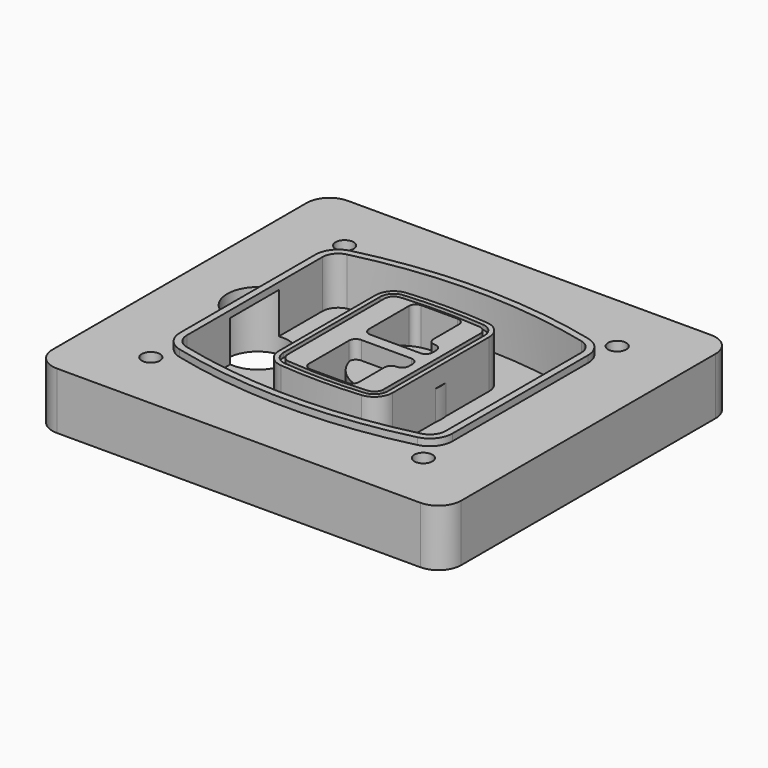
from build123d import *

# Parameters (mm, degrees)
F0_R      = 4
F1_DEPTH  = 25
F2_DEPTH  = 3
F3_DEPTH  = 18
F5_DEPTH  = 21
F6_DEPTH  = 2
F8_DEPTH  = 20
F9_DEPTH  = 16
F10_DEPTH = 25
F7_R      = 6
F7_R_2    = 4
F11_DEPTH = 6


# Not quite as in the source:
# - a feature of the source that left no trace in its solid (it failed there, or was rolled back) is left out


with BuildPart() as f1:
    # F0 (on Top) → F1 (new body)
    with BuildSketch(Plane.XY):
        with BuildLine():
            ThreePointArc((-90, -70), (-87.0710678119, -77.0710678119), (-80, -80))
            Line((-80, -80), (80, -80))
            ThreePointArc((80, -80), (87.0710678119, -77.0710678119), (90, -70))
            Line((90, -70), (90, 70))
            ThreePointArc((90, 70), (87.0710678119, 77.0710678119), (80, 80))
            Line((80, 80), (-80, 80))
            ThreePointArc((-80, 80), (-87.0710678119, 77.0710678119), (-90, 70))
            Line((-90, 70), (-90, -70))
        make_face()
        with Locations((-60, -53.3333333333)):
            Circle(F0_R, mode=Mode.SUBTRACT)
        with Locations((60, -53.3333333333)):
            Circle(F0_R, mode=Mode.SUBTRACT)
        with Locations((-60, 53.3333333333)):
            Circle(F0_R, mode=Mode.SUBTRACT)
        with BuildLine():
            ThreePointArc((-64, 37.2990447398), (-61.0143011354, 45.9411029726), (-53.3306899286, 50.8970778549))
            ThreePointArc((-53.3306899286, 50.8970778549), (0, 57.3333333333), (53.3306899286, 50.8970778549))
            ThreePointArc((53.3306899286, 50.8970778549), (61.0143011354, 45.9411029726), (64, 37.2990447398))
            Line((64, 37.2990447398), (64, -37.2990447398))
            ThreePointArc((64, -37.2990447398), (61.0143011354, -45.9411029726), (53.3306899286, -50.8970778549))
            ThreePointArc((53.3306899286, -50.8970778549), (0, -57.3333333333), (-53.3306899286, -50.8970778549))
            ThreePointArc((-53.3306899286, -50.8970778549), (-61.0143011354, -45.9411029726), (-64, -37.2990447398))
            Line((-64, -37.2990447398), (-64, 37.2990447398))
        make_face(mode=Mode.SUBTRACT)
        with Locations((60, 53.3333333333)):
            Circle(F0_R, mode=Mode.SUBTRACT)
        with BuildLine():
            ThreePointArc((53.3306899286, 50.8970778549), (0, 57.3333333333), (-53.3306899286, 50.8970778549))
            ThreePointArc((-53.3306899286, 50.8970778549), (-61.0143011354, 45.9411029726), (-64, 37.2990447398))
            Line((-64, 37.2990447398), (-64, -37.2990447398))
            ThreePointArc((-64, -37.2990447398), (-61.0143011354, -45.9411029726), (-53.3306899286, -50.8970778549))
            ThreePointArc((-53.3306899286, -50.8970778549), (0, -57.3333333333), (53.3306899286, -50.8970778549))
            ThreePointArc((53.3306899286, -50.8970778549), (61.0143011354, -45.9411029726), (64, -37.2990447398))
            Line((64, -37.2990447398), (64, 37.2990447398))
            ThreePointArc((64, 37.2990447398), (61.0143011354, 45.9411029726), (53.3306899286, 50.8970778549))
        make_face()
        with BuildLine():
            Line((-60, -37.2990447398), (-60, 37.2990447398))
            ThreePointArc((-60, 37.2990447398), (-57.8673579538, 43.4719434775), (-52.3790642347, 47.0119255363))
            ThreePointArc((-52.3790642347, 47.0119255363), (0, 53.3333333333), (52.3790642347, 47.0119255363))
            ThreePointArc((52.3790642347, 47.0119255363), (57.8673579538, 43.4719434775), (60, 37.2990447398))
            Line((60, 37.2990447398), (60, -37.2990447398))
            ThreePointArc((60, -37.2990447398), (57.8673579538, -43.4719434775), (52.3790642347, -47.0119255363))
            ThreePointArc((52.3790642347, -47.0119255363), (0, -53.3333333333), (-52.3790642347, -47.0119255363))
            ThreePointArc((-52.3790642347, -47.0119255363), (-57.8673579538, -43.4719434775), (-60, -37.2990447398))
        make_face(mode=Mode.SUBTRACT)
        with BuildLine():
            ThreePointArc((-52.3790642347, 47.0119255363), (-57.8673579538, 43.4719434775), (-60, 37.2990447398))
            Line((-60, 37.2990447398), (-60, -37.2990447398))
            ThreePointArc((-60, -37.2990447398), (-57.8673579538, -43.4719434775), (-52.3790642347, -47.0119255363))
            ThreePointArc((-52.3790642347, -47.0119255363), (0, -53.3333333333), (52.3790642347, -47.0119255363))
            ThreePointArc((52.3790642347, -47.0119255363), (57.8673579538, -43.4719434775), (60, -37.2990447398))
            Line((60, -37.2990447398), (60, 37.2990447398))
            ThreePointArc((60, 37.2990447398), (57.8673579538, 43.4719434775), (52.3790642347, 47.0119255363))
            ThreePointArc((52.3790642347, 47.0119255363), (0, 53.3333333333), (-52.3790642347, 47.0119255363))
        make_face()
        with BuildLine():
            ThreePointArc((51.6653449643, 44.0980612973), (55.5071505677, 41.6200738562), (57, 37.2990447398))
            Line((57, 37.2990447398), (57, -37.2990447398))
            ThreePointArc((57, -37.2990447398), (55.5071505677, -41.6200738562), (51.6653449643, -44.0980612973))
            ThreePointArc((51.6653449643, -44.0980612973), (0, -50.3333333333), (-51.6653449643, -44.0980612973))
            ThreePointArc((-51.6653449643, -44.0980612973), (-55.5071505677, -41.6200738562), (-57, -37.2990447398))
            Line((-57, -37.2990447398), (-57, 37.2990447398))
            ThreePointArc((-57, 37.2990447398), (-55.5071505677, 41.6200738562), (-51.6653449643, 44.0980612973))
            ThreePointArc((-51.6653449643, 44.0980612973), (0, 50.3333333333), (51.6653449643, 44.0980612973))
        make_face(mode=Mode.SUBTRACT)
        with BuildLine():
            Line((57, -37.2990447398), (57, 37.2990447398))
            ThreePointArc((57, 37.2990447398), (55.5071505677, 41.6200738562), (51.6653449643, 44.0980612973))
            ThreePointArc((51.6653449643, 44.0980612973), (0, 50.3333333333), (-51.6653449643, 44.0980612973))
            ThreePointArc((-51.6653449643, 44.0980612973), (-55.5071505677, 41.6200738562), (-57, 37.2990447398))
            Line((-57, 37.2990447398), (-57, -37.2990447398))
            ThreePointArc((-57, -37.2990447398), (-55.5071505677, -41.6200738562), (-51.6653449643, -44.0980612973))
            ThreePointArc((-51.6653449643, -44.0980612973), (0, -50.3333333333), (51.6653449643, -44.0980612973))
            ThreePointArc((51.6653449643, -44.0980612973), (55.5071505677, -41.6200738562), (57, -37.2990447398))
        make_face()
    extrude(amount=-F1_DEPTH)

    # F0 (on Top) → F2 (join)
    with BuildSketch(Plane.XY):
        with BuildLine():
            ThreePointArc((-52.3790642347, 47.0119255363), (-57.8673579538, 43.4719434775), (-60, 37.2990447398))
            Line((-60, 37.2990447398), (-60, -37.2990447398))
            ThreePointArc((-60, -37.2990447398), (-57.8673579538, -43.4719434775), (-52.3790642347, -47.0119255363))
            ThreePointArc((-52.3790642347, -47.0119255363), (0, -53.3333333333), (52.3790642347, -47.0119255363))
            ThreePointArc((52.3790642347, -47.0119255363), (57.8673579538, -43.4719434775), (60, -37.2990447398))
            Line((60, -37.2990447398), (60, 37.2990447398))
            ThreePointArc((60, 37.2990447398), (57.8673579538, 43.4719434775), (52.3790642347, 47.0119255363))
            ThreePointArc((52.3790642347, 47.0119255363), (0, 53.3333333333), (-52.3790642347, 47.0119255363))
        make_face()
        with BuildLine():
            ThreePointArc((51.6653449643, 44.0980612973), (55.5071505677, 41.6200738562), (57, 37.2990447398))
            Line((57, 37.2990447398), (57, -37.2990447398))
            ThreePointArc((57, -37.2990447398), (55.5071505677, -41.6200738562), (51.6653449643, -44.0980612973))
            ThreePointArc((51.6653449643, -44.0980612973), (0, -50.3333333333), (-51.6653449643, -44.0980612973))
            ThreePointArc((-51.6653449643, -44.0980612973), (-55.5071505677, -41.6200738562), (-57, -37.2990447398))
            Line((-57, -37.2990447398), (-57, 37.2990447398))
            ThreePointArc((-57, 37.2990447398), (-55.5071505677, 41.6200738562), (-51.6653449643, 44.0980612973))
            ThreePointArc((-51.6653449643, 44.0980612973), (0, 50.3333333333), (51.6653449643, 44.0980612973))
        make_face(mode=Mode.SUBTRACT)
    extrude(amount=F2_DEPTH)

    # F0 (on Top) → F3 (cut)
    with BuildSketch(Plane.XY):
        with BuildLine():
            Line((57, -37.2990447398), (57, 37.2990447398))
            ThreePointArc((57, 37.2990447398), (55.5071505677, 41.6200738562), (51.6653449643, 44.0980612973))
            ThreePointArc((51.6653449643, 44.0980612973), (0, 50.3333333333), (-51.6653449643, 44.0980612973))
            ThreePointArc((-51.6653449643, 44.0980612973), (-55.5071505677, 41.6200738562), (-57, 37.2990447398))
            Line((-57, 37.2990447398), (-57, -37.2990447398))
            ThreePointArc((-57, -37.2990447398), (-55.5071505677, -41.6200738562), (-51.6653449643, -44.0980612973))
            ThreePointArc((-51.6653449643, -44.0980612973), (0, -50.3333333333), (51.6653449643, -44.0980612973))
            ThreePointArc((51.6653449643, -44.0980612973), (55.5071505677, -41.6200738562), (57, -37.2990447398))
        make_face()
    extrude(amount=-F3_DEPTH, mode=Mode.SUBTRACT)

    # F4 (on face) → F5 (join, through all)
    with BuildSketch(Plane.XY.offset(3)):
        with BuildLine():
            ThreePointArc((-25, -26.587695628), (-22.8992979869, -31.9912392117), (-17.7004291845, -34.5569740744))
            ThreePointArc((-17.7004291845, -34.5569740744), (0, -35.3333333333), (17.7004291845, -34.5569740744))
            ThreePointArc((17.7004291845, -34.5569740744), (22.8992979869, -31.9912392117), (25, -26.587695628))
            Line((25, -26.587695628), (25, 26.587695628))
            ThreePointArc((25, 26.587695628), (22.8992979869, 31.9912392117), (17.7004291845, 34.5569740744))
            ThreePointArc((17.7004291845, 34.5569740744), (0, 35.3333333333), (-17.7004291845, 34.5569740744))
            ThreePointArc((-17.7004291845, 34.5569740744), (-22.8992979869, 31.9912392117), (-25, 26.587695628))
            Line((-25, 26.587695628), (-25, -26.587695628))
        make_face()
        with BuildLine():
            ThreePointArc((17.5253218884, 32.5646544628), (21.4244734902, 30.6403533158), (23, 26.587695628))
            Line((23, 26.587695628), (23, -26.587695628))
            ThreePointArc((23, -26.587695628), (21.4244734902, -30.6403533158), (17.5253218884, -32.5646544628))
            ThreePointArc((17.5253218884, -32.5646544628), (0, -33.3333333333), (-17.5253218884, -32.5646544628))
            ThreePointArc((-17.5253218884, -32.5646544628), (-21.4244734902, -30.6403533158), (-23, -26.587695628))
            Line((-23, -26.587695628), (-23, 26.587695628))
            ThreePointArc((-23, 26.587695628), (-21.4244734902, 30.6403533158), (-17.5253218884, 32.5646544628))
            ThreePointArc((-17.5253218884, 32.5646544628), (0, 33.3333333333), (17.5253218884, 32.5646544628))
        make_face(mode=Mode.SUBTRACT)
        with BuildLine():
            Line((23, -26.587695628), (23, 26.587695628))
            ThreePointArc((23, 26.587695628), (21.4244734902, 30.6403533158), (17.5253218884, 32.5646544628))
            ThreePointArc((17.5253218884, 32.5646544628), (0, 33.3333333333), (-17.5253218884, 32.5646544628))
            ThreePointArc((-17.5253218884, 32.5646544628), (-21.4244734902, 30.6403533158), (-23, 26.587695628))
            Line((-23, 26.587695628), (-23, -26.587695628))
            ThreePointArc((-23, -26.587695628), (-21.4244734902, -30.6403533158), (-17.5253218884, -32.5646544628))
            ThreePointArc((-17.5253218884, -32.5646544628), (0, -33.3333333333), (17.5253218884, -32.5646544628))
            ThreePointArc((17.5253218884, -32.5646544628), (21.4244734902, -30.6403533158), (23, -26.587695628))
        make_face()
        with BuildLine():
            ThreePointArc((17.3502145923, 30.5723348512), (19.9496489934, 29.2894674198), (21, 26.587695628))
            Line((21, 26.587695628), (21, -26.587695628))
            ThreePointArc((21, -26.587695628), (19.9496489934, -29.2894674198), (17.3502145923, -30.5723348512))
            ThreePointArc((17.3502145923, -30.5723348512), (0, -31.3333333333), (-17.3502145923, -30.5723348512))
            ThreePointArc((-17.3502145923, -30.5723348512), (-19.9496489934, -29.2894674198), (-21, -26.587695628))
            Line((-21, -26.587695628), (-21, 26.587695628))
            ThreePointArc((-21, 26.587695628), (-19.9496489934, 29.2894674198), (-17.3502145923, 30.5723348512))
            ThreePointArc((-17.3502145923, 30.5723348512), (0, 31.3333333333), (17.3502145923, 30.5723348512))
        make_face(mode=Mode.SUBTRACT)
        with BuildLine():
            Line((21, -26.587695628), (21, 26.587695628))
            ThreePointArc((21, 26.587695628), (19.9496489934, 29.2894674198), (17.3502145923, 30.5723348512))
            ThreePointArc((17.3502145923, 30.5723348512), (0, 31.3333333333), (-17.3502145923, 30.5723348512))
            ThreePointArc((-17.3502145923, 30.5723348512), (-19.9496489934, 29.2894674198), (-21, 26.587695628))
            Line((-21, 26.587695628), (-21, -26.587695628))
            ThreePointArc((-21, -26.587695628), (-19.9496489934, -29.2894674198), (-17.3502145923, -30.5723348512))
            ThreePointArc((-17.3502145923, -30.5723348512), (0, -31.3333333333), (17.3502145923, -30.5723348512))
            ThreePointArc((17.3502145923, -30.5723348512), (19.9496489934, -29.2894674198), (21, -26.587695628))
        make_face()
        with BuildLine():
            Line((-8, -2.5), (14, -2.5))
            ThreePointArc((14, -2.5), (16.1213203436, -3.3786796564), (17, -5.5))
            Line((17, -5.5), (17, -7.5))
            ThreePointArc((17, -7.5), (16.1213203436, -9.6213203436), (14, -10.5))
            ThreePointArc((14, -10.5), (11.8786796564, -11.3786796564), (11, -13.5))
            Line((11, -13.5), (11, -27.5))
            ThreePointArc((11, -27.5), (10.1213203436, -29.6213203436), (8, -30.5))
            Line((8, -30.5), (-8, -30.5))
            ThreePointArc((-8, -30.5), (-10.1213203436, -29.6213203436), (-11, -27.5))
            Line((-11, -27.5), (-11, -5.5))
            ThreePointArc((-11, -5.5), (-10.1213203436, -3.3786796564), (-8, -2.5))
        make_face(mode=Mode.SUBTRACT)
        with BuildLine():
            ThreePointArc((-8, 2.5), (-10.1213203436, 3.3786796564), (-11, 5.5))
            Line((-11, 5.5), (-11, 27.5))
            ThreePointArc((-11, 27.5), (-10.1213203436, 29.6213203436), (-8, 30.5))
            Line((-8, 30.5), (8, 30.5))
            ThreePointArc((8, 30.5), (10.1213203436, 29.6213203436), (11, 27.5))
            Line((11, 27.5), (11, 13.5))
            ThreePointArc((11, 13.5), (11.8786796564, 11.3786796564), (14, 10.5))
            ThreePointArc((14, 10.5), (16.1213203436, 9.6213203436), (17, 7.5))
            Line((17, 7.5), (17, 5.5))
            ThreePointArc((17, 5.5), (16.1213203436, 3.3786796564), (14, 2.5))
            Line((14, 2.5), (-8, 2.5))
        make_face(mode=Mode.SUBTRACT)
    extrude(amount=-F5_DEPTH)

    # F4 (on face) → F6 (cut)
    with BuildSketch(Plane.XY.offset(3)):
        with BuildLine():
            Line((23, -26.587695628), (23, 26.587695628))
            ThreePointArc((23, 26.587695628), (21.4244734902, 30.6403533158), (17.5253218884, 32.5646544628))
            ThreePointArc((17.5253218884, 32.5646544628), (0, 33.3333333333), (-17.5253218884, 32.5646544628))
            ThreePointArc((-17.5253218884, 32.5646544628), (-21.4244734902, 30.6403533158), (-23, 26.587695628))
            Line((-23, 26.587695628), (-23, -26.587695628))
            ThreePointArc((-23, -26.587695628), (-21.4244734902, -30.6403533158), (-17.5253218884, -32.5646544628))
            ThreePointArc((-17.5253218884, -32.5646544628), (0, -33.3333333333), (17.5253218884, -32.5646544628))
            ThreePointArc((17.5253218884, -32.5646544628), (21.4244734902, -30.6403533158), (23, -26.587695628))
        make_face()
        with BuildLine():
            ThreePointArc((17.3502145923, 30.5723348512), (19.9496489934, 29.2894674198), (21, 26.587695628))
            Line((21, 26.587695628), (21, -26.587695628))
            ThreePointArc((21, -26.587695628), (19.9496489934, -29.2894674198), (17.3502145923, -30.5723348512))
            ThreePointArc((17.3502145923, -30.5723348512), (0, -31.3333333333), (-17.3502145923, -30.5723348512))
            ThreePointArc((-17.3502145923, -30.5723348512), (-19.9496489934, -29.2894674198), (-21, -26.587695628))
            Line((-21, -26.587695628), (-21, 26.587695628))
            ThreePointArc((-21, 26.587695628), (-19.9496489934, 29.2894674198), (-17.3502145923, 30.5723348512))
            ThreePointArc((-17.3502145923, 30.5723348512), (0, 31.3333333333), (17.3502145923, 30.5723348512))
        make_face(mode=Mode.SUBTRACT)
    extrude(amount=-F6_DEPTH, mode=Mode.SUBTRACT)

    # F7 (on face) → F8 (join)
    with BuildSketch(Plane(origin=(0, 0, -25), x_dir=(1, 0, 0), z_dir=(0, 0, -1))):
        with BuildLine():
            ThreePointArc((-6.71157564, 0), (6.7567035675, 13.4682792075), (20.224982775, 0))
            Line((20.224982775, 0), (25.224982775, 0))
            ThreePointArc((25.224982775, 0), (6.7567035675, 18.4682792075), (-11.71157564, 0))
            Line((-11.71157564, 0), (-6.71157564, 0))
        make_face()
        with BuildLine():
            Line((-6.71157564, 0), (20.224982775, 0))
            ThreePointArc((20.224982775, 0), (6.7567035675, 13.4682792075), (-6.71157564, 0))
        make_face()
        with BuildLine():
            ThreePointArc((-6.71157564, 0), (6.7567035675, -13.4682792075), (20.224982775, 0))
            Line((20.224982775, 0), (-6.71157564, 0))
        make_face()
        with BuildLine():
            Line((25.224982775, 0), (20.224982775, 0))
            ThreePointArc((20.224982775, 0), (6.7567035675, -13.4682792075), (-6.71157564, 0))
            Line((-6.71157564, 0), (-11.71157564, 0))
            ThreePointArc((-11.71157564, 0), (6.7567035675, -18.4682792075), (25.224982775, 0))
        make_face()
    extrude(amount=-F8_DEPTH)

    # F7 (on face) → F9 (cut)
    with BuildSketch(Plane(origin=(0, 0, -25), x_dir=(1, 0, 0), z_dir=(0, 0, -1))):
        with BuildLine():
            Line((-6.71157564, 0), (20.224982775, 0))
            ThreePointArc((20.224982775, 0), (6.7567035675, 13.4682792075), (-6.71157564, 0))
        make_face()
        with BuildLine():
            ThreePointArc((-6.71157564, 0), (6.7567035675, -13.4682792075), (20.224982775, 0))
            Line((20.224982775, 0), (-6.71157564, 0))
        make_face()
    extrude(amount=-F9_DEPTH, mode=Mode.SUBTRACT)

    # F7 (on face) → F10 (cut)
    with BuildSketch(Plane(origin=(0, 0, -25), x_dir=(1, 0, 0), z_dir=(0, 0, -1))):
        with BuildLine():
            Line((-69.0318229325, 0), (-42.0952645175, 0))
            ThreePointArc((-42.0952645175, 0), (-55.563543725, 13.4682792075), (-69.0318229325, 0))
        make_face()
        with BuildLine():
            ThreePointArc((-69.0318229325, 0), (-55.563543725, -13.4682792075), (-42.0952645175, 0))
            Line((-42.0952645175, 0), (-69.0318229325, 0))
        make_face()
    extrude(amount=-F10_DEPTH, mode=Mode.SUBTRACT)

    # F7 (on face) → F11 (cut)
    with BuildSketch(Plane(origin=(0, 0, -25), x_dir=(1, 0, 0), z_dir=(0, 0, -1))):
        with Locations((60, -53.3333333333)):
            Circle(F7_R)
        with Locations((60, -53.3333333333)):
            Circle(F7_R_2, mode=Mode.SUBTRACT)
        with Locations((-60, -53.3333333333)):
            Circle(F7_R)
        with Locations((-60, -53.3333333333)):
            Circle(F7_R_2, mode=Mode.SUBTRACT)
        with Locations((-60, 53.3333333333)):
            Circle(F7_R)
        with Locations((-60, 53.3333333333)):
            Circle(F7_R_2, mode=Mode.SUBTRACT)
        with Locations((60, 53.3333333333)):
            Circle(F7_R)
        with Locations((60, 53.3333333333)):
            Circle(F7_R_2, mode=Mode.SUBTRACT)
    extrude(amount=-F11_DEPTH, mode=Mode.SUBTRACT)


solid = f1.part
